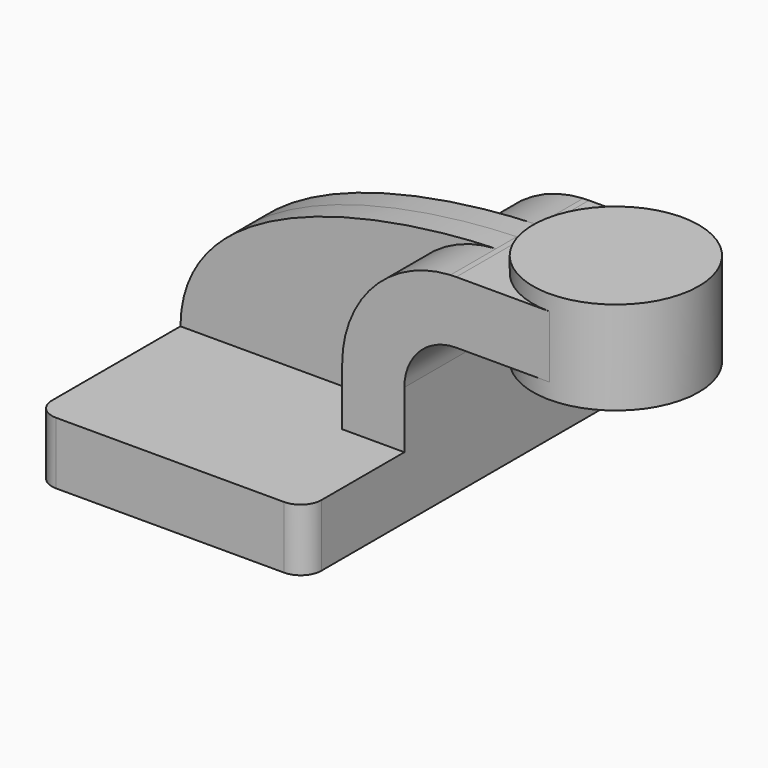
from build123d import *

# Parameters (mm, degrees)
F1_DEPTH = 63.5
F2_DEPTH = 25.4
F3_DEPTH = 7.9375
F5_R     = 6.35


# Not quite as in the source:
# - a feature names something its author has since deleted; it is built from what else it names


with BuildPart() as f1:
    # F0 (on Front) → F1 (new body, symmetric)
    with BuildSketch(Plane.XZ):
        Polygon((41.275, -9.525), (41.275, 9.525), (22.225, 9.525), (-41.275, 9.525), (-41.275, -9.525), align=None)
    extrude(amount=F1_DEPTH, both=True)

    # F0 (on Front) → F2 (join, symmetric)
    with BuildSketch(Plane.XZ):
        with BuildLine():
            Line((22.225, 9.525), (41.275, 9.525))
            Line((41.275, 9.525), (41.275, 27.0002))
            ThreePointArc((41.275, 27.0002), (45.9246798487, 38.2255201513), (57.15, 42.8752))
            Line((57.15, 42.8752), (60.325, 42.8752))
            Line((60.325, 42.8752), (60.325, 61.9252))
            Line((60.325, 61.9252), (57.15, 61.9252))
            add(Edge.make_bspline(
                [(55.3844542669, 61.8805450852), (55.9790813374, 61.8982519362), (56.5677127817, 61.9131134827), (57.15, 61.9252)],
                knots=[109.7272835167, 109.7272835167, 109.7272835167, 109.7272835167, 111.5045361635, 111.5045361635, 111.5045361635, 111.5045361635], degree=3))
            ThreePointArc((55.3844542669, 61.8805450852), (31.8377765721, 51.0635948173), (22.225, 27.0002))
            Line((22.225, 27.0002), (22.225, 9.525))
        make_face()
        Polygon((60.325, 61.9252), (60.325, 42.8752), (71.4375, 42.8752), (85.725, 42.8752), (85.725, 61.9252), (71.4375, 61.9252), align=None)
    extrude(amount=F2_DEPTH, both=True)

    # F0 (on Front) → F3 (join, symmetric)
    with BuildSketch(Plane.XZ):
        with BuildLine():
            Line((-41.275, 9.525), (22.225, 9.525))
            Line((22.225, 9.525), (22.225, 27.0002))
            ThreePointArc((22.225, 27.0002), (31.8377765721, 51.0635948173), (55.3844542669, 61.8805450852))
            add(Edge.make_bspline(
                [(-41.275, 9.525), (-40.8940696255, 48.8483570296), (18.6722776014, 60.7873270442), (55.3844542669, 61.8805450852)],
                knots=[0, 0, 0, 0, 109.7272835167, 109.7272835167, 109.7272835167, 109.7272835167], degree=3))
        make_face()
    extrude(amount=F3_DEPTH, both=True)

    # F0 (on Front) → F4 (revolve)
    with BuildSketch(Plane.XZ):
        Polygon((85.725, 42.8752), (85.725, 38.1), (111.125, 38.1), (111.125, 66.675), (85.725, 66.675), (85.725, 61.9252), align=None)
    revolve(axis=Axis((85.725, 0, 52.4002), (0, 0, 1)))

    # F5
    f5_edges = [f1.edges().sort_by_distance(p)[0] for p in [
        (-41.275, -63.5, 0),
        (41.275, -63.5, 0),
        (41.275, 63.5, 0),
        (-41.275, 63.5, 0),
    ]]
    fillet(f5_edges, radius=F5_R)


solid = f1.part
